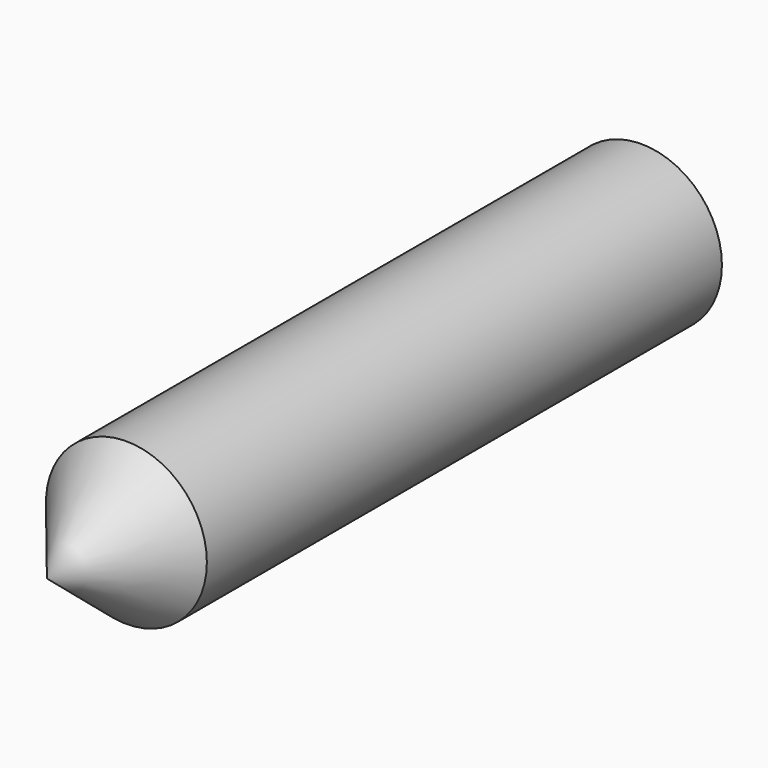
from build123d import *

# Parameters (mm, degrees)
F0_R     = 19.05
F0_R_2   = 12.7
F1_DEPTH = 152.4
F2_R     = 19.05


# Not quite as in the source:
# - an extrude whose draft closes it to a point is written as a loft to that point


with BuildPart() as f1:
    # F0 (on Front) → F1 (new body)
    with BuildSketch(Plane.XZ):
        Circle(F0_R)
        Circle(F0_R_2, mode=Mode.SUBTRACT)
    extrude(amount=F1_DEPTH)

    # F2 (on face) → F3 section 0
    with BuildSketch(Plane.XZ.offset(152.4), mode=Mode.PRIVATE) as f3_s0:
        Circle(F2_R)
    loft([f3_s0.sketch, Vertex(0, -175.924790832, 0)], ruled=True)


solid = f1.part
